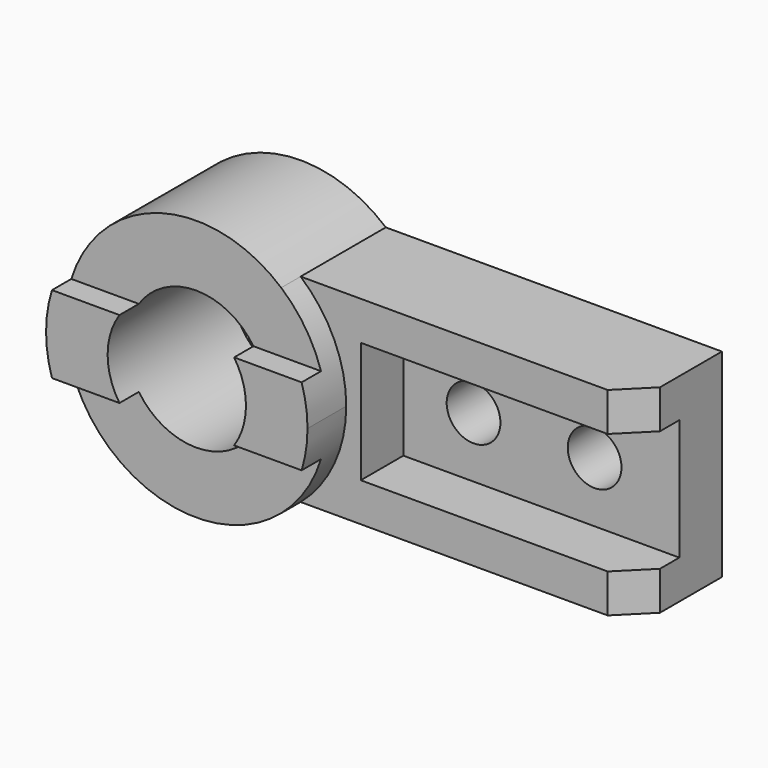
from build123d import *

# Parameters (mm, degrees)
F0_R     = 11.1
F1_DEPTH = 44
F0_R_2   = 28.575
F2_DEPTH = 64
F4_DEPTH = 95.001
F5_W     = 114
F5_H     = 50
F6_DEPTH = 22
F8_DEPTH = 10


with BuildPart() as f1:
    # F0 (on Front) → F1 (new body)
    with BuildSketch(Plane.XZ):
        with BuildLine():
            ThreePointArc((35.1425667816, 41), (49.0596504584, 22.5643678594), (54, 0))
            ThreePointArc((54, 0), (49.0596504584, -22.5643678594), (35.1425667816, -41))
            Line((35.1425667816, -41), (174, -41))
            Line((174, -41), (174, 41))
            Line((174, 41), (35.1425667816, 41))
        make_face()
        with Locations((89, 0)):
            Circle(F0_R, mode=Mode.SUBTRACT)
        with Locations((139, 0)):
            Circle(F0_R, mode=Mode.SUBTRACT)
    extrude(amount=F1_DEPTH)

    # F0 (on Front) → F2 (join)
    with BuildSketch(Plane.XZ):
        with BuildLine():
            ThreePointArc((35.1425667816, -41), (49.0596504584, -22.5643678594), (54, 0))
            ThreePointArc((54, 0), (49.0596504584, 22.5643678594), (35.1425667816, 41))
            ThreePointArc((35.1425667816, 41), (-54, 0), (35.1425667816, -41))
        make_face()
        Circle(F0_R_2, mode=Mode.SUBTRACT)
    extrude(amount=F2_DEPTH)

    # F3 (on face) → F4 (cut, through all)
    with BuildSketch(Plane.XY.offset(41)):
        Polygon((174, -44), (174, -32), (162, -44), align=None)
    extrude(amount=-F4_DEPTH, mode=Mode.SUBTRACT)

    # F5 (on face) → F6 (cut)
    with BuildSketch(Plane.XZ.offset(44)):
        with Locations((117, 0)):
            Rectangle(F5_W, F5_H)
    extrude(amount=-F6_DEPTH, mode=Mode.SUBTRACT)

    # F7 (on face) → F8 (cut)
    with BuildSketch(Plane.XZ.offset(64)):
        with BuildLine():
            ThreePointArc((51.5751878329, 16), (0, 54), (-51.5751878329, 16))
            Line((-51.5751878329, 16), (-23.6755279772, 16))
            ThreePointArc((-23.6755279772, 16), (0, 28.575), (23.6755279772, 16))
            Line((23.6755279772, 16), (51.5751878329, 16))
        make_face()
        with BuildLine():
            Line((-23.6755279772, -16), (-51.5751878329, -16))
            ThreePointArc((-51.5751878329, -16), (0, -54), (51.5751878329, -16))
            Line((51.5751878329, -16), (23.6755279772, -16))
            ThreePointArc((23.6755279772, -16), (0, -28.575), (-23.6755279772, -16))
        make_face()
    extrude(amount=-F8_DEPTH, mode=Mode.SUBTRACT)


solid = f1.part
